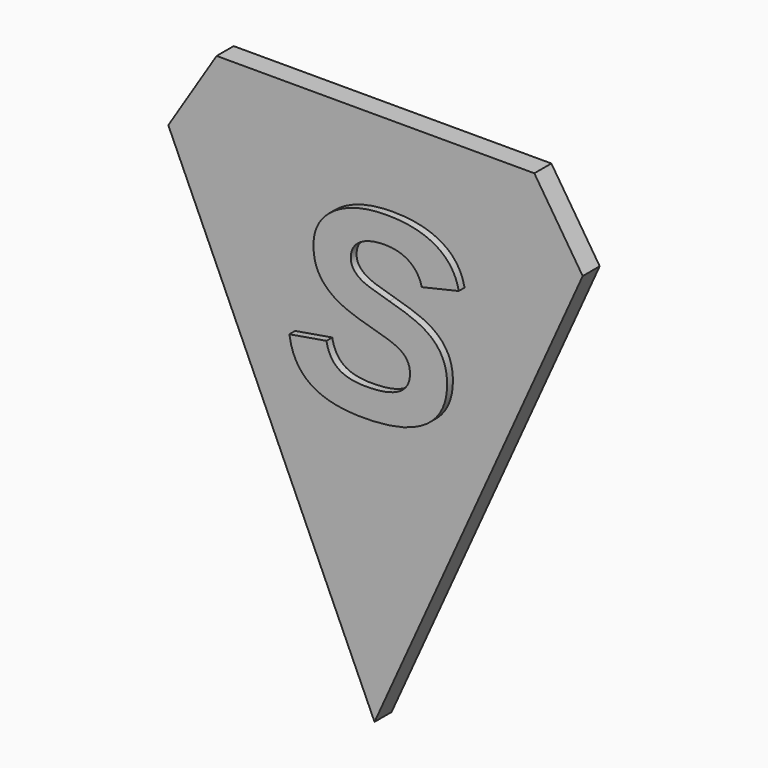
from build123d import *

# Parameters (mm, degrees)
F1_DEPTH     = 2.5
F2_TEXT_SIZE = 61.7675405617
F3_DEPTH     = 1.7


# Not quite as in the source:
# - Text() gives the source's letters only with a copy of the font that has no kerning and outlines rounded to 1/6400 em; it was checked with that copy


with BuildPart() as f1:
    # F0 (on Front) → F1 (new body, symmetric)
    with BuildSketch(Plane.XZ):
        Polygon((25.442307815, 31.8777449429), (14.0841379762, 49.4450516999), (-60.5769231915, 49.4450516999), (-71.935094893, 31.423419714), (-23.4735589474, -76.2674510479), align=None)
    extrude(amount=F1_DEPTH, both=True)

    # F2 (on face) → F3 (join, symmetric)
    with BuildSketch(Plane.XZ.offset(2.5)):
        with Locations((-42.8843256086, -12.459021993)):
            Text('S', F2_TEXT_SIZE, font='Arimo', font_style=FontStyle.BOLDITALIC, text_align=(TextAlign.LEFT, TextAlign.BOTTOM))
    extrude(amount=F3_DEPTH, both=True)


solid = f1.part
